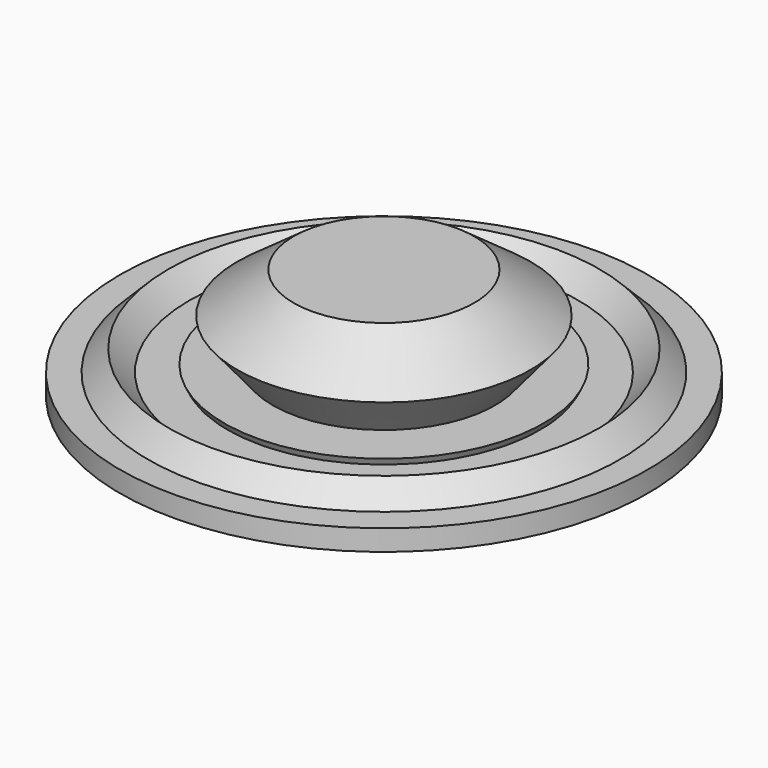
from build123d import *

# Parameters (mm, degrees)
F5_DEPTH = 1.5


with BuildPart() as f1:
    # F0 (on Front) → F1 (revolve)
    with BuildSketch(Plane.XZ):
        with BuildLine():
            Line((-11.5, 2), (-10.5, 0))
            Line((-10.5, 0), (-5, 0))
            Line((-5, 0), (-5, 5))
            ThreePointArc((-5, 5), (-4.7071067812, 5.7071067812), (-4, 6))
            Line((-4, 6), (0, 6))
            Line((0, 6), (0, 8))
            Line((0, 8), (-6.5, 8))
            Line((-6.5, 8), (-10.5563024928, 5.0765756232))
            Line((-10.5563024928, 5.0765756232), (-8, 2))
            Line((-8, 2), (-11.5, 2))
        make_face()
    revolve(axis=Axis((0, 0, 7), (0, 0, -1)))


with BuildPart() as f3:
    # F2 (on Front) → F3 (revolve)
    with BuildSketch(Plane.XZ):
        Polygon((-19, 1.5), (-19, 0), (-11, 0), (-11, 1.5), (-14, 1.5), (-15.500000224, 3), (-17, 1.5), align=None)
    revolve(axis=Axis((0, 0, 1.6170465387), (0, 0, 1)))

    # F4 (on face) → F5 (join, through all)
    with BuildSketch(Plane(origin=(0, 0, 0), x_dir=(1, 0, 0), z_dir=(0, 0, -1))):
        with BuildLine():
            ThreePointArc((2, 10.8166538264), (0, 11), (-2, 10.8166538264))
            ThreePointArc((-2, 10.8166538264), (0, 10), (2, 10.8166538264))
        make_face()
        with BuildLine():
            ThreePointArc((-8.3674969976, -7.1403777208), (-8.6602540378, -5), (-10.3674969976, -3.6762761056))
            ThreePointArc((-10.3674969976, -3.6762761056), (-9.5262794416, -5.5), (-8.3674969976, -7.1403777208))
        make_face()
        with BuildLine():
            ThreePointArc((8.3674969976, -7.1403777208), (9.5262794416, -5.5), (10.3674969976, -3.6762761056))
            ThreePointArc((10.3674969976, -3.6762761056), (8.6602540378, -5), (8.3674969976, -7.1403777208))
        make_face()
    extrude(amount=-F5_DEPTH)


solid = Compound([f1.part, f3.part])
